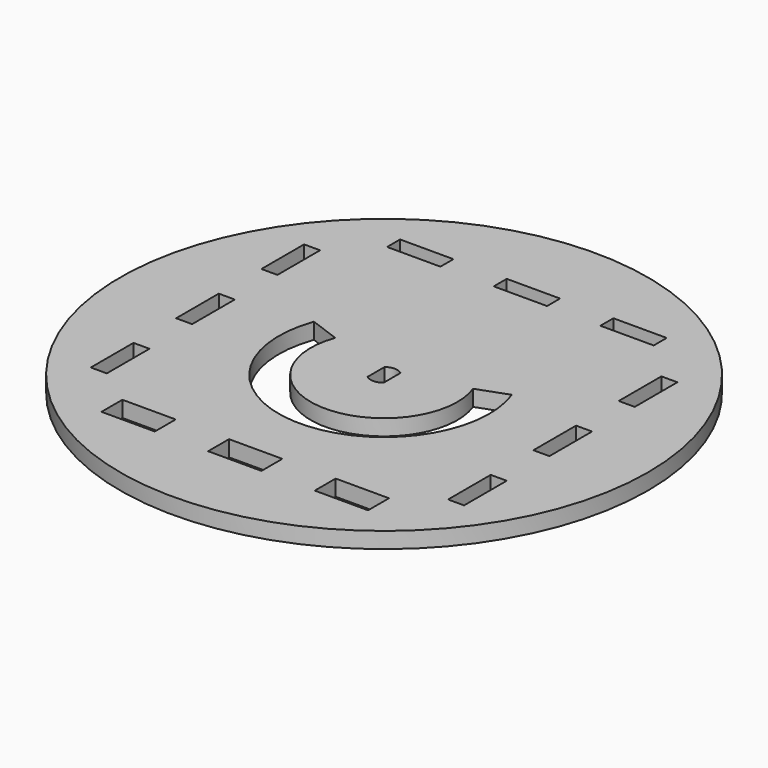
from build123d import *

# Parameters (mm, degrees)
F0_R     = 49.4974746831
F0_W     = 10
F0_H     = 4.9
F0_W_2   = 3
F0_H_2   = 10
F0_H_3   = 3.05
F1_DEPTH = 3


with BuildPart() as f1:
    # F0 (on Top) → F1 (new body)
    with BuildSketch(Plane.XY):
        Circle(F0_R)
        with Locations((-19.9997237325, -32.55)):
            Rectangle(F0_W, F0_H, mode=Mode.SUBTRACT)
        with Locations((-33.5, -20)):
            Rectangle(F0_W_2, F0_H_2, mode=Mode.SUBTRACT)
        with Locations((0.0002762675, -32.55)):
            Rectangle(F0_W, F0_H, mode=Mode.SUBTRACT)
        with Locations((20.0002762675, -32.55)):
            Rectangle(F0_W, F0_H, mode=Mode.SUBTRACT)
        with BuildLine():
            ThreePointArc((18.5589292605, 6.7548978307), (0, -19.75), (-18.5589292605, 6.7548978307))
            Line((-18.5589292605, 6.7548978307), (-12.9207735358, 4.7027769707))
            ThreePointArc((-12.9207735358, 4.7027769707), (0, -13.75), (12.9207735358, 4.7027769707))
            Line((12.9207735358, 4.7027769707), (18.5589292605, 6.7548978307))
        make_face(mode=Mode.SUBTRACT)
        with Locations((33.5, -20)):
            Rectangle(F0_W_2, F0_H_2, mode=Mode.SUBTRACT)
        with Locations((-33.5, 0)):
            Rectangle(F0_W_2, F0_H_2, mode=Mode.SUBTRACT)
        with Locations((-33.5, 20)):
            Rectangle(F0_W_2, F0_H_2, mode=Mode.SUBTRACT)
        with Locations((-20, 33.475)):
            Rectangle(F0_W, F0_H_3, mode=Mode.SUBTRACT)
        with BuildLine():
            ThreePointArc((-1.5, 2), (0, 2.5), (1.5, 2))
            Line((1.5, 2), (1.5, -2))
            ThreePointArc((1.5, -2), (0, -2.5), (-1.5, -2))
            Line((-1.5, -2), (-1.5, 2))
        make_face(mode=Mode.SUBTRACT)
        with Locations((33.5, 0)):
            Rectangle(F0_W_2, F0_H_2, mode=Mode.SUBTRACT)
        with Locations((33.5, 20)):
            Rectangle(F0_W_2, F0_H_2, mode=Mode.SUBTRACT)
        with Locations((0, 33.475)):
            Rectangle(F0_W, F0_H_3, mode=Mode.SUBTRACT)
        with Locations((20, 33.475)):
            Rectangle(F0_W, F0_H_3, mode=Mode.SUBTRACT)
    extrude(amount=F1_DEPTH)


solid = f1.part
